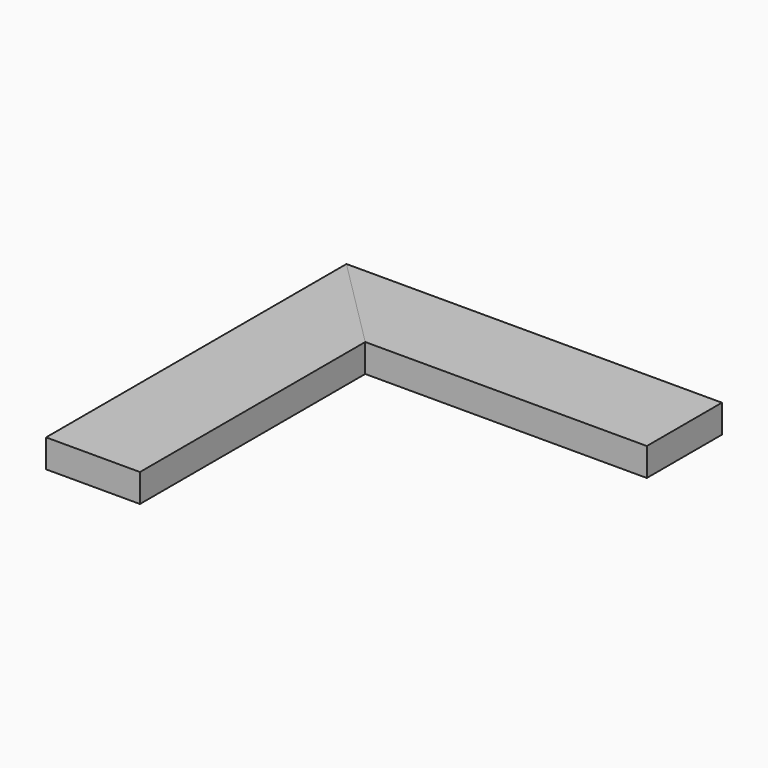
from build123d import *

# Parameters (mm, degrees)
F2_DEPTH = 19.05
F4_DEPTH = 9.525
F5_W     = 254
F5_H     = 63.5
F6_DEPTH = 19.05


# Not quite as in the source:
# - a variable given as a bare number and used for a length is read in inches; the dataset says mm whatever the document's units were


with BuildPart() as f2:
    # F1 (on Top) → F2 (new body)
    with BuildSketch(Plane.XY):
        Polygon((0, 254), (0, 0), (63.5, 0), (63.5, 190.5), align=None)
    extrude(amount=F2_DEPTH)

    # F3 (on face) → F4 (join)
    with BuildSketch(Plane(origin=(0, 0, 0), x_dir=(1, 0, 0), z_dir=(0, 0, -1))):
        with BuildLine():
            ThreePointArc((40.8742306969, -220.7908973636), (33.3906839294, -223.8906839294), (30.2908973636, -231.3742306969))
            ThreePointArc((30.2908973636, -231.3742306969), (40.8742306969, -241.9575640303), (51.4575640303, -231.3742306969))
            ThreePointArc((51.4575640303, -231.3742306969), (48.3577774645, -223.8906839294), (40.8742306969, -220.7908973636))
        make_face()
        with BuildLine():
            ThreePointArc((24.8708333161, -229.1291666839), (28.3309172501, -228.4409131765), (30.2908973636, -231.3742306969))
            ThreePointArc((30.2908973636, -231.3742306969), (33.3906839294, -223.8906839294), (40.8742306969, -220.7908973636))
            ThreePointArc((40.8742306969, -220.7908973636), (37.9409131848, -218.83091727), (38.6291666535, -215.3708333465))
            Line((38.6291666535, -215.3708333465), (24.8708333161, -229.1291666839))
        make_face()
    extrude(amount=-F4_DEPTH)


with BuildPart() as f6:
    # F5 (on Top) → F6 (new body)
    with BuildSketch(Plane.XY):
        with Locations((127, 222.25)):
            Rectangle(F5_W, F5_H)
    extrude(amount=F6_DEPTH)

    # F7: cut F2
    add(f2.part, mode=Mode.SUBTRACT)


solid = Compound([f2.part, f6.part])
